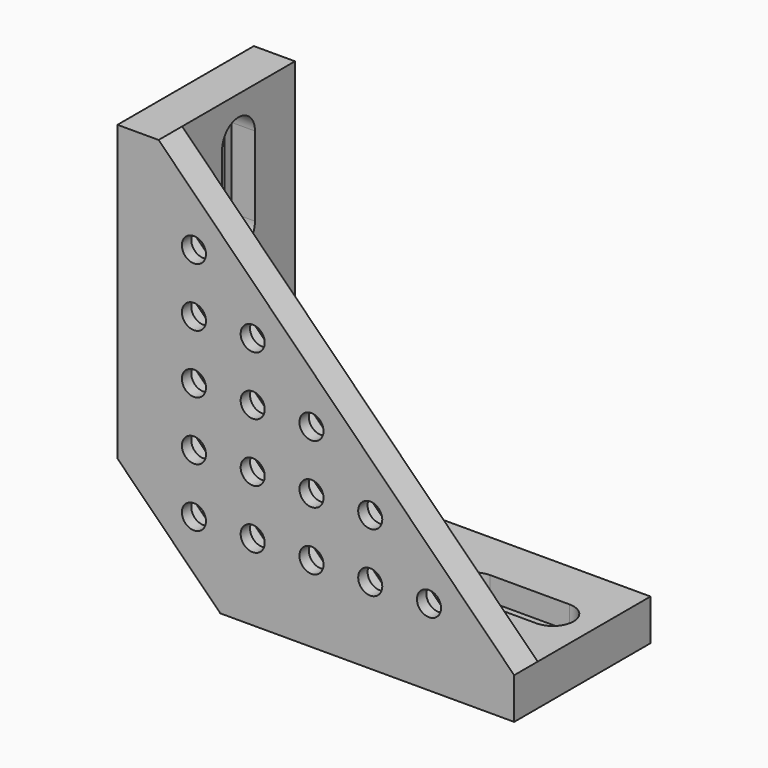
from build123d import *

# Parameters (mm, degrees)
F1_DEPTH  = 7
F2_DEPTH  = 3
F4_ANGLE  = 90
F8_ANGLE  = 180
F12_R     = 2.05
F13_DEPTH = 5
F14_DEPTH = 3


# Not quite as in the source:
# - a feature names something its author has since deleted; it is built from what else it names


with BuildPart() as f1:
    # F0 (on Top) → F1 (new body)
    with BuildSketch(Plane.XY):
        Polygon((29, 12), (-21, 12), (-21, -12), (0, -12), (29, -12), align=None)
        with BuildLine():
            ThreePointArc((-14, -11.5), (-17.5, -8), (-14, -4.5))
            Line((-14, -4.5), (2, -4.5))
            Line((2, -4.5), (22, -4.5))
            ThreePointArc((22, -4.5), (25.5, -8), (22, -11.5))
            Line((22, -11.5), (2, -11.5))
            Line((2, -11.5), (-14, -11.5))
        make_face(mode=Mode.SUBTRACT)
        with BuildLine():
            Line((-0.5, -3.5), (-14, -3.5))
            ThreePointArc((-14, -3.5), (-17.5, 0), (-14, 3.5))
            Line((-14, 3.5), (-0.5, 3.5))
            Line((-0.5, 3.5), (2, 3.5))
            Line((2, 3.5), (8.5, 3.5))
            Line((8.5, 3.5), (22, 3.5))
            ThreePointArc((22, 3.5), (25.5, 0), (22, -3.5))
            Line((22, -3.5), (8.5, -3.5))
            Line((8.5, -3.5), (2, -3.5))
            Line((2, -3.5), (-0.5, -3.5))
        make_face(mode=Mode.SUBTRACT)
        with BuildLine():
            Line((0, 4.5), (-14, 4.5))
            ThreePointArc((-14, 4.5), (-17.5, 8), (-14, 11.5))
            Line((-14, 11.5), (0, 11.5))
            Line((0, 11.5), (22, 11.5))
            ThreePointArc((22, 11.5), (25.5, 8), (22, 4.5))
            Line((22, 4.5), (0, 4.5))
        make_face(mode=Mode.SUBTRACT)
        with BuildLine():
            Line((2, -4.5), (-14, -4.5))
            ThreePointArc((-14, -4.5), (-17.5, -8), (-14, -11.5))
            Line((-14, -11.5), (2, -11.5))
            Line((2, -11.5), (22, -11.5))
            ThreePointArc((22, -11.5), (25.5, -8), (22, -4.5))
            Line((22, -4.5), (2, -4.5))
        make_face()
        with BuildLine():
            ThreePointArc((-14, -10.05), (-16.05, -8), (-14, -5.95))
            Line((-14, -5.95), (0, -5.95))
            Line((0, -5.95), (22, -5.95))
            ThreePointArc((22, -5.95), (24.05, -8), (22, -10.05))
            Line((22, -10.05), (0, -10.05))
            Line((0, -10.05), (-14, -10.05))
        make_face(mode=Mode.SUBTRACT)
        with BuildLine():
            ThreePointArc((-14, 11.5), (-17.5, 8), (-14, 4.5))
            Line((-14, 4.5), (0, 4.5))
            Line((0, 4.5), (22, 4.5))
            ThreePointArc((22, 4.5), (25.5, 8), (22, 11.5))
            Line((22, 11.5), (0, 11.5))
            Line((0, 11.5), (-14, 11.5))
        make_face()
        with BuildLine():
            Line((22, 5.95), (0, 5.95))
            Line((0, 5.95), (-14, 5.95))
            ThreePointArc((-14, 5.95), (-16.05, 8), (-14, 10.05))
            Line((-14, 10.05), (0, 10.05))
            Line((0, 10.05), (22, 10.05))
            ThreePointArc((22, 10.05), (24.05, 8), (22, 5.95))
        make_face(mode=Mode.SUBTRACT)
        with BuildLine():
            Line((0, -5.95), (-14, -5.95))
            ThreePointArc((-14, -5.95), (-16.05, -8), (-14, -10.05))
            Line((-14, -10.05), (0, -10.05))
            Line((0, -10.05), (22, -10.05))
            ThreePointArc((22, -10.05), (24.05, -8), (22, -5.95))
            Line((22, -5.95), (0, -5.95))
        make_face()
        with BuildLine():
            Line((-14, 5.95), (0, 5.95))
            Line((0, 5.95), (22, 5.95))
            ThreePointArc((22, 5.95), (24.05, 8), (22, 10.05))
            Line((22, 10.05), (0, 10.05))
            Line((0, 10.05), (-14, 10.05))
            ThreePointArc((-14, 10.05), (-16.05, 8), (-14, 5.95))
        make_face()
        with BuildLine():
            ThreePointArc((-0.5, 3.5), (3, 0), (-0.5, -3.5))
            Line((-0.5, -3.5), (2, -3.5))
            Line((2, -3.5), (8.5, -3.5))
            ThreePointArc((8.5, -3.5), (5, 0), (8.5, 3.5))
            Line((8.5, 3.5), (2, 3.5))
            Line((2, 3.5), (-0.5, 3.5))
        make_face()
    extrude(amount=F1_DEPTH)

    # F0 (on Top) → F2 (join)
    with BuildSketch(Plane.XY):
        with BuildLine():
            ThreePointArc((-14, 3.5), (-17.5, 0), (-14, -3.5))
            Line((-14, -3.5), (-0.5, -3.5))
            ThreePointArc((-0.5, -3.5), (3, 0), (-0.5, 3.5))
            Line((-0.5, 3.5), (-14, 3.5))
        make_face()
        with BuildLine():
            Line((-0.5, -2.05), (-14, -2.05))
            ThreePointArc((-14, -2.05), (-16.05, 0), (-14, 2.05))
            Line((-14, 2.05), (-0.5, 2.05))
            ThreePointArc((-0.5, 2.05), (1.55, 0), (-0.5, -2.05))
        make_face(mode=Mode.SUBTRACT)
        with BuildLine():
            ThreePointArc((8.5, 3.5), (5, 0), (8.5, -3.5))
            Line((8.5, -3.5), (22, -3.5))
            ThreePointArc((22, -3.5), (25.5, 0), (22, 3.5))
            Line((22, 3.5), (8.5, 3.5))
        make_face()
        with BuildLine():
            ThreePointArc((22, 2.05), (24.05, 0), (22, -2.05))
            Line((22, -2.05), (8.5, -2.05))
            ThreePointArc((8.5, -2.05), (6.45, 0), (8.5, 2.05))
            Line((8.5, 2.05), (22, 2.05))
        make_face(mode=Mode.SUBTRACT)
    extrude(amount=F2_DEPTH)


with BuildPart() as f4_1:
    # F4: copy of F1
    add(f1.part.rotate(Axis((-21, 0, 3.5), (0, -1, 0)), F4_ANGLE))


with BuildPart() as f4_1_1:
    # F8: moved
    add(f4_1.part.rotate(Axis((-21, 0, 28.5), (0, 0, 1)), F8_ANGLE))


with BuildPart() as f4_1_2:
    # F9: moved
    add(f4_1_1.part.moved(Location((0, 0, 14))))


with BuildPart() as f4_1_3:
    # F10: moved
    add(f4_1_2.part.moved(Location((-14, 0, 0))))


with BuildPart() as f1_1:
    add(f1.part)

    add(f4_1_3.part)  # F13 merges F4_1
    # F12 (on 3pt) → F13 (join)
    with BuildSketch(Plane.XZ.offset(12)):
        Polygon((-38.5, 17.5), (-21, 0), (29, 0), (29, 7), (-31.5, 67.5), (-38.5, 67.5), align=None)
        Polygon((-29.3563439923, 11.9720831325), (-28.3210678119, 15.8357864376), (-24.4573645067, 16.871062618), (-21.628937382, 14.0426354933), (-22.6642135624, 10.1789321881), (-26.5279168675, 9.1436560077), align=None, mode=Mode.SUBTRACT)
        Polygon((-19.3563439923, 11.9720831325), (-18.3210678119, 15.8357864376), (-14.4573645067, 16.871062618), (-11.628937382, 14.0426354933), (-12.6642135624, 10.1789321881), (-16.5279168675, 9.1436560077), align=None, mode=Mode.SUBTRACT)
        Polygon((-9.3563439923, 11.9720831325), (-8.3210678119, 15.8357864376), (-4.4573645067, 16.871062618), (-1.628937382, 14.0426354933), (-2.6642135624, 10.1789321881), (-6.5279168675, 9.1436560077), align=None, mode=Mode.SUBTRACT)
        Polygon((-29.3563439923, 21.9720831325), (-28.3210678119, 25.8357864376), (-24.4573645067, 26.871062618), (-21.628937382, 24.0426354933), (-22.6642135624, 20.1789321881), (-26.5279168675, 19.1436560077), align=None, mode=Mode.SUBTRACT)
        Polygon((-29.3563439923, 31.9720831325), (-28.3210678119, 35.8357864376), (-24.4573645067, 36.871062618), (-21.628937382, 34.0426354933), (-22.6642135624, 30.1789321881), (-26.5279168675, 29.1436560077), align=None, mode=Mode.SUBTRACT)
        Polygon((-19.3563439923, 21.9720831325), (-18.3210678119, 25.8357864376), (-14.4573645067, 26.871062618), (-11.628937382, 24.0426354933), (-12.6642135624, 20.1789321881), (-16.5279168675, 19.1436560077), align=None, mode=Mode.SUBTRACT)
        Polygon((-9.3563439923, 21.9720831325), (-8.3210678119, 25.8357864376), (-4.4573645067, 26.871062618), (-1.628937382, 24.0426354933), (-2.6642135624, 20.1789321881), (-6.5279168675, 19.1436560077), align=None, mode=Mode.SUBTRACT)
        Polygon((-19.3563439923, 31.9720831325), (-18.3210678119, 35.8357864376), (-14.4573645067, 36.871062618), (-11.628937382, 34.0426354933), (-12.6642135624, 30.1789321881), (-16.5279168675, 29.1436560077), align=None, mode=Mode.SUBTRACT)
        Polygon((-9.3563439923, 31.9720831325), (-8.3210678119, 35.8357864376), (-4.4573645067, 36.871062618), (-1.628937382, 34.0426354933), (-2.6642135624, 30.1789321881), (-6.5279168675, 29.1436560077), align=None, mode=Mode.SUBTRACT)
        Polygon((0.6436560077, 11.9720831325), (1.6789321881, 15.8357864376), (5.5426354933, 16.871062618), (8.371062618, 14.0426354933), (7.3357864376, 10.1789321881), (3.4720831325, 9.1436560077), align=None, mode=Mode.SUBTRACT)
        Polygon((10.6436560077, 11.9720831325), (11.6789321881, 15.8357864376), (15.5426354933, 16.871062618), (18.371062618, 14.0426354933), (17.3357864376, 10.1789321881), (13.4720831325, 9.1436560077), align=None, mode=Mode.SUBTRACT)
        Polygon((0.6436560077, 21.9720831325), (1.6789321881, 25.8357864376), (5.5426354933, 26.871062618), (8.371062618, 24.0426354933), (7.3357864376, 20.1789321881), (3.4720831325, 19.1436560077), align=None, mode=Mode.SUBTRACT)
        Polygon((-29.3563439923, 41.9720831325), (-28.3210678119, 45.8357864376), (-24.4573645067, 46.871062618), (-21.628937382, 44.0426354933), (-22.6642135624, 40.1789321881), (-26.5279168675, 39.1436560077), align=None, mode=Mode.SUBTRACT)
        Polygon((-19.3563439923, 41.9720831325), (-18.3210678119, 45.8357864376), (-14.4573645067, 46.871062618), (-11.628937382, 44.0426354933), (-12.6642135624, 40.1789321881), (-16.5279168675, 39.1436560077), align=None, mode=Mode.SUBTRACT)
        Polygon((-26.5279168675, 49.1436560077), (-29.3563439923, 51.9720831325), (-28.3210678119, 55.8357864376), (-24.4573645067, 56.871062618), (-21.628937382, 54.0426354933), (-22.6642135624, 50.1789321881), align=None, mode=Mode.SUBTRACT)
        Polygon((-4.4573645067, 36.871062618), (-8.3210678119, 35.8357864376), (-9.3563439923, 31.9720831325), (-6.5279168675, 29.1436560077), (-2.6642135624, 30.1789321881), (-1.628937382, 34.0426354933), align=None)
        with Locations((-5.4926406871, 33.0073593129)):
            Circle(F12_R, mode=Mode.SUBTRACT)
        Polygon((-14.4573645067, 46.871062618), (-18.3210678119, 45.8357864376), (-19.3563439923, 41.9720831325), (-16.5279168675, 39.1436560077), (-12.6642135624, 40.1789321881), (-11.628937382, 44.0426354933), align=None)
        with Locations((-15.4926406871, 43.0073593129)):
            Circle(F12_R, mode=Mode.SUBTRACT)
        Polygon((-14.4573645067, 36.871062618), (-18.3210678119, 35.8357864376), (-19.3563439923, 31.9720831325), (-16.5279168675, 29.1436560077), (-12.6642135624, 30.1789321881), (-11.628937382, 34.0426354933), align=None)
        with Locations((-15.4926406871, 33.0073593129)):
            Circle(F12_R, mode=Mode.SUBTRACT)
        Polygon((-14.4573645067, 26.871062618), (-18.3210678119, 25.8357864376), (-19.3563439923, 21.9720831325), (-16.5279168675, 19.1436560077), (-12.6642135624, 20.1789321881), (-11.628937382, 24.0426354933), align=None)
        with Locations((-15.4926406871, 23.0073593129)):
            Circle(F12_R, mode=Mode.SUBTRACT)
        Polygon((-4.4573645067, 26.871062618), (-8.3210678119, 25.8357864376), (-9.3563439923, 21.9720831325), (-6.5279168675, 19.1436560077), (-2.6642135624, 20.1789321881), (-1.628937382, 24.0426354933), align=None)
        with Locations((-5.4926406871, 23.0073593129)):
            Circle(F12_R, mode=Mode.SUBTRACT)
        Polygon((5.5426354933, 26.871062618), (1.6789321881, 25.8357864376), (0.6436560077, 21.9720831325), (3.4720831325, 19.1436560077), (7.3357864376, 20.1789321881), (8.371062618, 24.0426354933), align=None)
        with Locations((4.5073593129, 23.0073593129)):
            Circle(F12_R, mode=Mode.SUBTRACT)
        Polygon((-28.3210678119, 55.8357864376), (-29.3563439923, 51.9720831325), (-26.5279168675, 49.1436560077), (-22.6642135624, 50.1789321881), (-21.628937382, 54.0426354933), (-24.4573645067, 56.871062618), align=None)
        with Locations((-25.4926406871, 53.0073593129)):
            Circle(F12_R, mode=Mode.SUBTRACT)
        Polygon((-24.4573645067, 46.871062618), (-28.3210678119, 45.8357864376), (-29.3563439923, 41.9720831325), (-26.5279168675, 39.1436560077), (-22.6642135624, 40.1789321881), (-21.628937382, 44.0426354933), align=None)
        with Locations((-25.4926406871, 43.0073593129)):
            Circle(F12_R, mode=Mode.SUBTRACT)
        Polygon((-24.4573645067, 36.871062618), (-28.3210678119, 35.8357864376), (-29.3563439923, 31.9720831325), (-26.5279168675, 29.1436560077), (-22.6642135624, 30.1789321881), (-21.628937382, 34.0426354933), align=None)
        with Locations((-25.4926406871, 33.0073593129)):
            Circle(F12_R, mode=Mode.SUBTRACT)
        Polygon((-24.4573645067, 26.871062618), (-28.3210678119, 25.8357864376), (-29.3563439923, 21.9720831325), (-26.5279168675, 19.1436560077), (-22.6642135624, 20.1789321881), (-21.628937382, 24.0426354933), align=None)
        with Locations((-25.4926406871, 23.0073593129)):
            Circle(F12_R, mode=Mode.SUBTRACT)
        Polygon((-24.4573645067, 16.871062618), (-28.3210678119, 15.8357864376), (-29.3563439923, 11.9720831325), (-26.5279168675, 9.1436560077), (-22.6642135624, 10.1789321881), (-21.628937382, 14.0426354933), align=None)
        with Locations((-25.4926406871, 13.0073593129)):
            Circle(F12_R, mode=Mode.SUBTRACT)
        Polygon((-14.4573645067, 16.871062618), (-18.3210678119, 15.8357864376), (-19.3563439923, 11.9720831325), (-16.5279168675, 9.1436560077), (-12.6642135624, 10.1789321881), (-11.628937382, 14.0426354933), align=None)
        with Locations((-15.4926406871, 13.0073593129)):
            Circle(F12_R, mode=Mode.SUBTRACT)
        Polygon((-4.4573645067, 16.871062618), (-8.3210678119, 15.8357864376), (-9.3563439923, 11.9720831325), (-6.5279168675, 9.1436560077), (-2.6642135624, 10.1789321881), (-1.628937382, 14.0426354933), align=None)
        with Locations((-5.4926406871, 13.0073593129)):
            Circle(F12_R, mode=Mode.SUBTRACT)
        Polygon((5.5426354933, 16.871062618), (1.6789321881, 15.8357864376), (0.6436560077, 11.9720831325), (3.4720831325, 9.1436560077), (7.3357864376, 10.1789321881), (8.371062618, 14.0426354933), align=None)
        with Locations((4.5073593129, 13.0073593129)):
            Circle(F12_R, mode=Mode.SUBTRACT)
        Polygon((15.5426354933, 16.871062618), (11.6789321881, 15.8357864376), (10.6436560077, 11.9720831325), (13.4720831325, 9.1436560077), (17.3357864376, 10.1789321881), (18.371062618, 14.0426354933), align=None)
        with Locations((14.5073593129, 13.0073593129)):
            Circle(F12_R, mode=Mode.SUBTRACT)
    extrude(amount=F13_DEPTH)

    # F12 (on 3pt) → F14 (cut)
    with BuildSketch(Plane.XZ.offset(12)):
        Polygon((-4.4573645067, 36.871062618), (-8.3210678119, 35.8357864376), (-9.3563439923, 31.9720831325), (-6.5279168675, 29.1436560077), (-2.6642135624, 30.1789321881), (-1.628937382, 34.0426354933), align=None)
        with Locations((-5.4926406871, 33.0073593129)):
            Circle(F12_R, mode=Mode.SUBTRACT)
        Polygon((5.5426354933, 26.871062618), (1.6789321881, 25.8357864376), (0.6436560077, 21.9720831325), (3.4720831325, 19.1436560077), (7.3357864376, 20.1789321881), (8.371062618, 24.0426354933), align=None)
        with Locations((4.5073593129, 23.0073593129)):
            Circle(F12_R, mode=Mode.SUBTRACT)
        Polygon((-4.4573645067, 26.871062618), (-8.3210678119, 25.8357864376), (-9.3563439923, 21.9720831325), (-6.5279168675, 19.1436560077), (-2.6642135624, 20.1789321881), (-1.628937382, 24.0426354933), align=None)
        with Locations((-5.4926406871, 23.0073593129)):
            Circle(F12_R, mode=Mode.SUBTRACT)
        Polygon((-14.4573645067, 26.871062618), (-18.3210678119, 25.8357864376), (-19.3563439923, 21.9720831325), (-16.5279168675, 19.1436560077), (-12.6642135624, 20.1789321881), (-11.628937382, 24.0426354933), align=None)
        with Locations((-15.4926406871, 23.0073593129)):
            Circle(F12_R, mode=Mode.SUBTRACT)
        Polygon((-14.4573645067, 36.871062618), (-18.3210678119, 35.8357864376), (-19.3563439923, 31.9720831325), (-16.5279168675, 29.1436560077), (-12.6642135624, 30.1789321881), (-11.628937382, 34.0426354933), align=None)
        with Locations((-15.4926406871, 33.0073593129)):
            Circle(F12_R, mode=Mode.SUBTRACT)
        Polygon((-14.4573645067, 46.871062618), (-18.3210678119, 45.8357864376), (-19.3563439923, 41.9720831325), (-16.5279168675, 39.1436560077), (-12.6642135624, 40.1789321881), (-11.628937382, 44.0426354933), align=None)
        with Locations((-15.4926406871, 43.0073593129)):
            Circle(F12_R, mode=Mode.SUBTRACT)
        Polygon((15.5426354933, 16.871062618), (11.6789321881, 15.8357864376), (10.6436560077, 11.9720831325), (13.4720831325, 9.1436560077), (17.3357864376, 10.1789321881), (18.371062618, 14.0426354933), align=None)
        with Locations((14.5073593129, 13.0073593129)):
            Circle(F12_R, mode=Mode.SUBTRACT)
        Polygon((5.5426354933, 16.871062618), (1.6789321881, 15.8357864376), (0.6436560077, 11.9720831325), (3.4720831325, 9.1436560077), (7.3357864376, 10.1789321881), (8.371062618, 14.0426354933), align=None)
        with Locations((4.5073593129, 13.0073593129)):
            Circle(F12_R, mode=Mode.SUBTRACT)
        Polygon((-4.4573645067, 16.871062618), (-8.3210678119, 15.8357864376), (-9.3563439923, 11.9720831325), (-6.5279168675, 9.1436560077), (-2.6642135624, 10.1789321881), (-1.628937382, 14.0426354933), align=None)
        with Locations((-5.4926406871, 13.0073593129)):
            Circle(F12_R, mode=Mode.SUBTRACT)
        Polygon((-14.4573645067, 16.871062618), (-18.3210678119, 15.8357864376), (-19.3563439923, 11.9720831325), (-16.5279168675, 9.1436560077), (-12.6642135624, 10.1789321881), (-11.628937382, 14.0426354933), align=None)
        with Locations((-15.4926406871, 13.0073593129)):
            Circle(F12_R, mode=Mode.SUBTRACT)
        Polygon((-24.4573645067, 16.871062618), (-28.3210678119, 15.8357864376), (-29.3563439923, 11.9720831325), (-26.5279168675, 9.1436560077), (-22.6642135624, 10.1789321881), (-21.628937382, 14.0426354933), align=None)
        with Locations((-25.4926406871, 13.0073593129)):
            Circle(F12_R, mode=Mode.SUBTRACT)
        Polygon((-24.4573645067, 26.871062618), (-28.3210678119, 25.8357864376), (-29.3563439923, 21.9720831325), (-26.5279168675, 19.1436560077), (-22.6642135624, 20.1789321881), (-21.628937382, 24.0426354933), align=None)
        with Locations((-25.4926406871, 23.0073593129)):
            Circle(F12_R, mode=Mode.SUBTRACT)
        Polygon((-24.4573645067, 36.871062618), (-28.3210678119, 35.8357864376), (-29.3563439923, 31.9720831325), (-26.5279168675, 29.1436560077), (-22.6642135624, 30.1789321881), (-21.628937382, 34.0426354933), align=None)
        with Locations((-25.4926406871, 33.0073593129)):
            Circle(F12_R, mode=Mode.SUBTRACT)
        Polygon((-24.4573645067, 46.871062618), (-28.3210678119, 45.8357864376), (-29.3563439923, 41.9720831325), (-26.5279168675, 39.1436560077), (-22.6642135624, 40.1789321881), (-21.628937382, 44.0426354933), align=None)
        with Locations((-25.4926406871, 43.0073593129)):
            Circle(F12_R, mode=Mode.SUBTRACT)
        Polygon((-28.3210678119, 55.8357864376), (-29.3563439923, 51.9720831325), (-26.5279168675, 49.1436560077), (-22.6642135624, 50.1789321881), (-21.628937382, 54.0426354933), (-24.4573645067, 56.871062618), align=None)
        with Locations((-25.4926406871, 53.0073593129)):
            Circle(F12_R, mode=Mode.SUBTRACT)
    extrude(amount=F14_DEPTH, mode=Mode.SUBTRACT)


solid = f1_1.part
